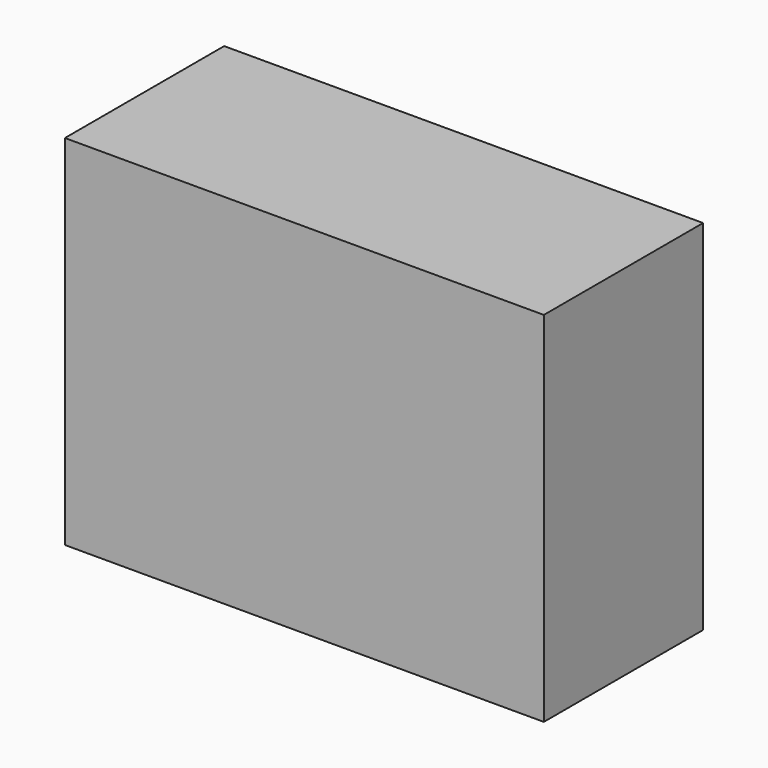
from build123d import *

# Parameters (mm, degrees)
F1_E0_BOTTOM_W = 305.5575340986
F1_E0_BOTTOM_H = 127
F2_DEPTH       = 228.6


with BuildPart() as f2:
    # F1_E0_bottom (on explicit) → F2 (new body)
    with BuildSketch(Plane(origin=(-118.9673468471, 0, 13.8002932072), x_dir=(1, 0, 0), z_dir=(0, 0, -1))):
        with Locations((152.7787670493, 63.5)):
            Rectangle(F1_E0_BOTTOM_W, F1_E0_BOTTOM_H)
    extrude(amount=F2_DEPTH)


solid = f2.part
